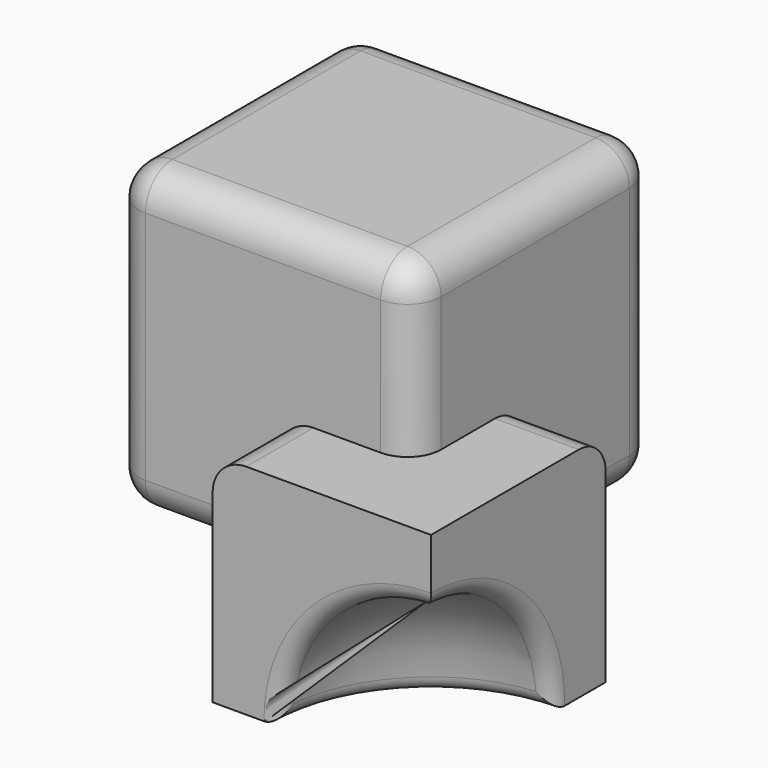
from build123d import *

# Parameters (mm, degrees)
F0_W         = 18
F0_H         = 18
F1_DEPTH     = 18
F2_W         = 10
F2_H         = 10
F2_W_2       = 3
F2_H_2       = 3
F3_DEPTH     = 5
F4_DEPTH     = 8
F5_R         = 2
F6_F1_R      = 2
F6_F2_R      = 2
F6_F3_R      = 2
F7_R         = 2
F11_T2_ANGLE = 120.2475861172
F11_T4_ANGLE = 120.2475861172
F11_T6_ANGLE = 120.2475861172


# Not quite as in the source:
# - a fillet or chamfer that OpenCascade refuses, or shapes differently, is made with other operations: its cross-section is extruded or revolved along the edge and cut away or added
# - two fillets or chamfers of one size are made in one step


with BuildPart() as f1:
    # F0 (on Front) → F1 (new body)
    with BuildSketch(Plane.XZ):
        with Locations((-9, 9)):
            Rectangle(F0_W, F0_H)
    extrude(amount=-F1_DEPTH)

    # F2 (on Top) → F3 (join)
    with BuildSketch(Plane.XY):
        Rectangle(F2_W, F2_H)
        with Locations((-6.5, 0)):
            Rectangle(F2_W_2, F2_H)
        with Locations((0, 6.5)):
            Rectangle(F2_W, F2_H_2)
        with Locations((-6.5, 6.5)):
            Rectangle(F2_W_2, F2_H_2)
    extrude(amount=-F3_DEPTH)

    # F2 (on Top) → F4 (join)
    with BuildSketch(Plane.XY):
        Rectangle(F2_W, F2_H)
        with Locations((-6.5, 0)):
            Rectangle(F2_W_2, F2_H)
        with Locations((0, 6.5)):
            Rectangle(F2_W, F2_H_2)
        with Locations((-6.5, 6.5)):
            Rectangle(F2_W_2, F2_H_2)
    extrude(amount=F4_DEPTH)

    # F5
    f5_edges = [f1.edges().sort_by_distance(p)[0] for p in [
        (-18, 18, 9),
        (-18, 9, 18),
        (-9, 18, 18),
    ]]
    fillet(f5_edges, radius=F5_R)

    # F6: fillet of radius 2 on 3 edges, made by hand

    # F6_f1
    f6_f1_edges = [f1.edges().sort_by_distance(p)[0] for p in [
        (-8, 18, 0),
        (-17.4142135624, 17.4142135624, 0),
        (-18, 8, 0),
    ]]
    fillet(f6_f1_edges, radius=F6_F1_R)

    # F6_f2
    f6_f2_edges = [f1.edges().sort_by_distance(p)[0] for p in [
        (0, 18, 9),
        (0, 8, 18),
        (0, 17.4142135624, 17.4142135624),
    ]]
    fillet(f6_f2_edges, radius=F6_F2_R)

    # F6_f3
    f6_f3_edges = [f1.edges().sort_by_distance(p)[0] for p in [
        (-18, 0, 9),
        (-17.4142135624, 0, 17.4142135624),
        (-9, 0, 18),
    ]]
    fillet(f6_f3_edges, radius=F6_F3_R)

    # F7
    f7_edges = [f1.edges().sort_by_distance(p)[0] for p in [
        (-8, -2.5, 8),
        (-8, 8, -2.5),
        (2.5, 8, 8),
    ]]
    fillet(f7_edges, radius=F7_R)

    # F9 (on face) → F10 (revolve, cut)
    with BuildSketch(Plane.XZ.offset(5)):
        with BuildLine():
            Line((5, -5), (5, 4))
            ThreePointArc((5, 4), (-1.3639610307, 1.3639610307), (-4, -5))
            Line((-4, -5), (5, -5))
        make_face()
    revolve(axis=Axis((5, -5, -0.5), (0, 0, -1)), mode=Mode.SUBTRACT)

    # F11: fillet of radius 1 on 3 edges, made by hand

    # F11_s1 → F11_t2 (revolve, cut)
    with BuildSketch(Plane(origin=(5.9189857789, 0, -1.5997021362), x_dir=(0, 1, 0), z_dir=(0.9653643687, 0, -0.2609054153))):
        with BuildLine():
            ThreePointArc((-5, 6.4275796043), (-4.7416198487, 5.756759211), (-4.1, 5.4325921672))
            ThreePointArc((-4.1, 5.4325921672), (-4.5494350245, 5.4664198912), (-5, 5.4777052332))
            Line((-5, 5.4777052332), (-5, 6.4275796043))
        make_face()
    revolve(axis=Axis((5, -5, -5), (0, -1, 0)), revolution_arc=F11_T2_ANGLE, mode=Mode.SUBTRACT)

    # F11_s3 → F11_t4 (revolve, cut)
    with BuildSketch(Plane(origin=(1.5997021362, -5.9189857789, 0), x_dir=(0, 0, 1), z_dir=(0.2609054153, -0.9653643687, 0))):
        with BuildLine():
            ThreePointArc((-5, 6.4275796043), (-4.7416198487, 5.756759211), (-4.1, 5.4325921672))
            ThreePointArc((-4.1, 5.4325921672), (-4.5494350245, 5.4664198912), (-5, 5.4777052332))
            Line((-5, 5.4777052332), (-5, 6.4275796043))
        make_face()
    revolve(axis=Axis((5, -5, -5), (0, 0, -1)), revolution_arc=F11_T4_ANGLE, mode=Mode.SUBTRACT)

    # F11_s5 → F11_t6 (revolve, cut)
    with BuildSketch(Plane(origin=(0, -1.5997021362, -5.9189857789), x_dir=(1, 0, 0), z_dir=(0, -0.2609054153, -0.9653643687))):
        with BuildLine():
            ThreePointArc((5, -6.4275796043), (4.7416198487, -5.756759211), (4.1, -5.4325921672))
            ThreePointArc((4.1, -5.4325921672), (4.5494350245, -5.4664198912), (5, -5.4777052332))
            Line((5, -5.4777052332), (5, -6.4275796043))
        make_face()
    revolve(axis=Axis((5, -5, -5), (1, 0, 0)), revolution_arc=F11_T6_ANGLE, mode=Mode.SUBTRACT)


solid = f1.part
